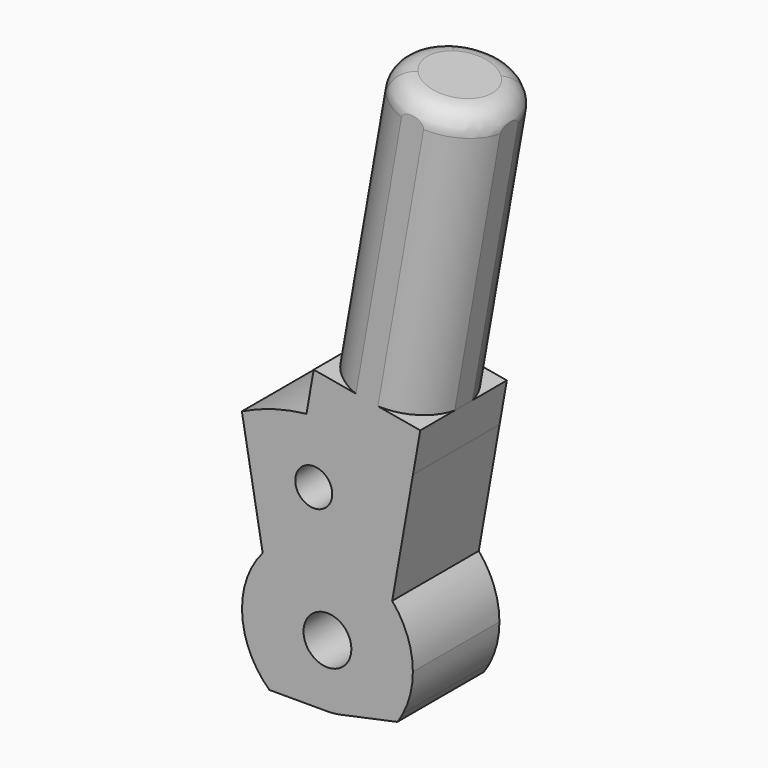
from build123d import *

# Parameters (mm, degrees)
F0_R        = 1.625
F0_R_2      = 2.1
F1_DEPTH    = 9.5
F3_DEPTH    = 25
F4_T2_ANGLE = 184.9085480034
F4_T4_ANGLE = 184.9085480034
F4_T6_ANGLE = 184.9085480034
F4_T8_ANGLE = 184.9085480034


# Not quite as in the source:
# - a fillet or chamfer that OpenCascade refuses, or shapes differently, is made with other operations: its cross-section is extruded or revolved along the edge and cut away or added
# - a feature names something its author has since deleted; it is built from what else it names


with BuildPart() as f1:
    # F0 (on Front) → F1 (new body)
    with BuildSketch(Plane.XZ):
        with BuildLine():
            Line((-7.512280983, 15.2501027679), (-5.6857070658, 4.891087319))
            ThreePointArc((-5.6857070658, 4.891087319), (0, 7.5), (5.6857070658, 4.891087319))
            Line((5.6857070658, 4.891087319), (7.512280983, 15.2501027679))
            Line((7.512280983, 15.2501027679), (8.1508003801, 18.8713262163))
            Line((8.1508003801, 18.8713262163), (-1.2048732735, 20.5209839042))
            Line((-1.2048732735, 20.5209839042), (-1.8433926706, 16.8997604558))
            ThreePointArc((-1.8433926706, 16.8997604558), (-4.75, 16.3229133429), (-7.512280983, 15.2501027679))
        make_face()
        with Locations((-1.2020773276, 11.4370017967)):
            Circle(F0_R, mode=Mode.SUBTRACT)
        with BuildLine():
            ThreePointArc((-5.6857070658, 4.891087319), (-7.452634421, 0.8415700723), (-6.6332495807, -3.5))
            Line((-6.6332495807, -3.5), (6.6332495807, -3.5))
            ThreePointArc((6.6332495807, -3.5), (7.2800883187, -1.8028627436), (7.5, 0))
            ThreePointArc((7.5, 0), (7.0318135283, 2.6083708523), (5.6857070658, 4.891087319))
            ThreePointArc((5.6857070658, 4.891087319), (0, 7.5), (-5.6857070658, 4.891087319))
        make_face()
        Circle(F0_R_2, mode=Mode.SUBTRACT)
        with BuildLine():
            ThreePointArc((-6.6332495807, -3.5), (-5.9507591554, -4.5649168092), (-5.0990195136, -5.5))
            Line((-5.0990195136, -5.5), (0, -5.5))
            ThreePointArc((0, -5.5), (0.574906548, -5.4698704245), (1.1435142995, -5.379811804))
            Line((1.1435142995, -5.379811804), (6.1311080028, -4.3196660355))
            ThreePointArc((6.1311080028, -4.3196660355), (6.3953240131, -3.9178860075), (6.6332495807, -3.5))
            Line((6.6332495807, -3.5), (-6.6332495807, -3.5))
        make_face()
    extrude(amount=F1_DEPTH)

    # F2 (on face) → F3 (join)
    with BuildSketch(Plane(origin=(3.4729635533, 0, 19.6961550602), x_dir=(0.984807753, 0, -0.1736481777), z_dir=(0.1736481777, 0, 0.984807753))):
        with BuildLine():
            Line((4.75, -5.7297958971), (4.75, -3.7702041029))
            ThreePointArc((4.75, -3.7702041029), (3.4294678888, -1.3205321112), (0.9797958971, 0))
            Line((0.9797958971, 0), (-0.9797958971, 0))
            ThreePointArc((-0.9797958971, 0), (-3.4294678888, -1.3205321112), (-4.75, -3.7702041029))
            Line((-4.75, -3.7702041029), (-4.75, -5.7297958971))
            ThreePointArc((-4.75, -5.7297958971), (-3.4294678888, -8.1794678888), (-0.9797958971, -9.5))
            Line((-0.9797958971, -9.5), (0.9797958971, -9.5))
            ThreePointArc((0.9797958971, -9.5), (3.4294678888, -8.1794678888), (4.75, -5.7297958971))
        make_face()
    extrude(amount=F3_DEPTH)

    # F4: fillet of radius 2 on 4 edges, made by hand

    # F4_s1 → F4_t2 (revolve, cut)
    with BuildSketch(Plane(origin=(2.3303405276, -2.5782182234, -0.4109019093), x_dir=(-0.7418696826, -0.6705440881, 0), z_dir=(-0.6659057216, 0.7367379343, 0.1174171453))):
        with BuildLine():
            ThreePointArc((2.4557468395, 43.6793554426), (1.6921353384, 45.0072275442), (0.2132331001, 45.4062200412))
            Line((0.2132331001, 45.4062200412), (0.187450643, 45.6046889581))
            ThreePointArc((0.187450643, 45.6046889581), (1.1796484238, 45.7331788115), (2.1717946748, 45.8620653318))
            Line((2.1717946748, 45.8620653318), (2.3960460488, 45.6893788719))
            ThreePointArc((2.3960460488, 45.6893788719), (2.5249325691, 44.6972326209), (2.6542157564, 43.7051378996))
            Line((2.6542157564, 43.7051378996), (2.4557468395, 43.6793554426))
        make_face()
    revolve(axis=Axis((7.814167995, -4.75, 44.3163488855), (0.1736481777, 0, 0.984807753)), revolution_arc=F4_T2_ANGLE, mode=Mode.SUBTRACT)

    # F4_s3 → F4_t4 (revolve, cut)
    with BuildSketch(Plane(origin=(-2.3303405276, -2.1717817766, 0.4109019093), x_dir=(0.6817807283, -0.731556586, 0), z_dir=(-0.7255452297, -0.6761783908, 0.1279331997))):
        with BuildLine():
            ThreePointArc((13.3818366305, 41.7080845524), (12.9673157833, 43.1827096947), (11.6314878435, 43.9323166305))
            Line((11.6314878435, 43.9323166305), (11.655182008, 44.1310456738))
            ThreePointArc((11.655182008, 44.1310456738), (12.6485812749, 44.0122013421), (13.6420278977, 43.8937541973))
            Line((13.6420278977, 43.8937541973), (13.8170627765, 43.6713309895))
            ThreePointArc((13.8170627765, 43.6713309895), (13.6986156317, 42.6778843667), (13.5805656738, 41.6843903878))
            Line((13.5805656738, 41.6843903878), (13.3818366305, 41.7080845524))
        make_face()
    revolve(axis=Axis((7.814167995, -4.75, 44.3163488855), (0.1736481777, 0, 0.984807753)), revolution_arc=F4_T4_ANGLE, mode=Mode.SUBTRACT)

    # F4_s5 → F4_t6 (revolve, cut)
    with BuildSketch(Plane(origin=(2.3303405276, -2.5782182234, -0.4109019093), x_dir=(0.7418696826, 0.6705440881, 0), z_dir=(0.6659057216, -0.7367379343, -0.1174171453))):
        with BuildLine():
            ThreePointArc((5.4373559827, 44.6721702336), (6.7652280844, 43.9085587325), (7.1642205814, 42.4296564942))
            Line((7.1642205814, 42.4296564942), (7.3626894983, 42.4038740371))
            ThreePointArc((7.3626894983, 42.4038740371), (7.4911793516, 43.3960718179), (7.6200658719, 44.3882180689))
            Line((7.6200658719, 44.3882180689), (7.4473794121, 44.6124694429))
            ThreePointArc((7.4473794121, 44.6124694429), (6.455233161, 44.7413559632), (5.4631384397, 44.8706391505))
            Line((5.4631384397, 44.8706391505), (5.4373559827, 44.6721702336))
        make_face()
    revolve(axis=Axis((7.814167995, -4.75, 44.3163488855), (0.1736481777, 0, 0.984807753)), revolution_arc=F4_T6_ANGLE, mode=Mode.SUBTRACT)

    # F4_s7 → F4_t8 (revolve, cut)
    with BuildSketch(Plane(origin=(-2.3303405276, -2.1717817766, 0.4109019093), x_dir=(-0.6817807283, 0.731556586, 0), z_dir=(0.7255452297, 0.6761783908, -0.1279331997))):
        with BuildLine():
            ThreePointArc((-5.9734927288, 44.6069108674), (-4.4988675865, 44.1923900202), (-3.7492606507, 42.8565620804))
            Line((-3.7492606507, 42.8565620804), (-3.5505316074, 42.880256245))
            ThreePointArc((-3.5505316074, 42.880256245), (-3.669375939, 43.8736555118), (-3.7878230838, 44.8671021347))
            Line((-3.7878230838, 44.8671021347), (-4.0102462916, 45.0421370134))
            ThreePointArc((-4.0102462916, 45.0421370134), (-5.0036929145, 44.9236898686), (-5.9971868933, 44.8056399107))
            Line((-5.9971868933, 44.8056399107), (-5.9734927288, 44.6069108674))
        make_face()
    revolve(axis=Axis((7.814167995, -4.75, 44.3163488855), (0.1736481777, 0, 0.984807753)), revolution_arc=F4_T8_ANGLE, mode=Mode.SUBTRACT)


solid = f1.part
